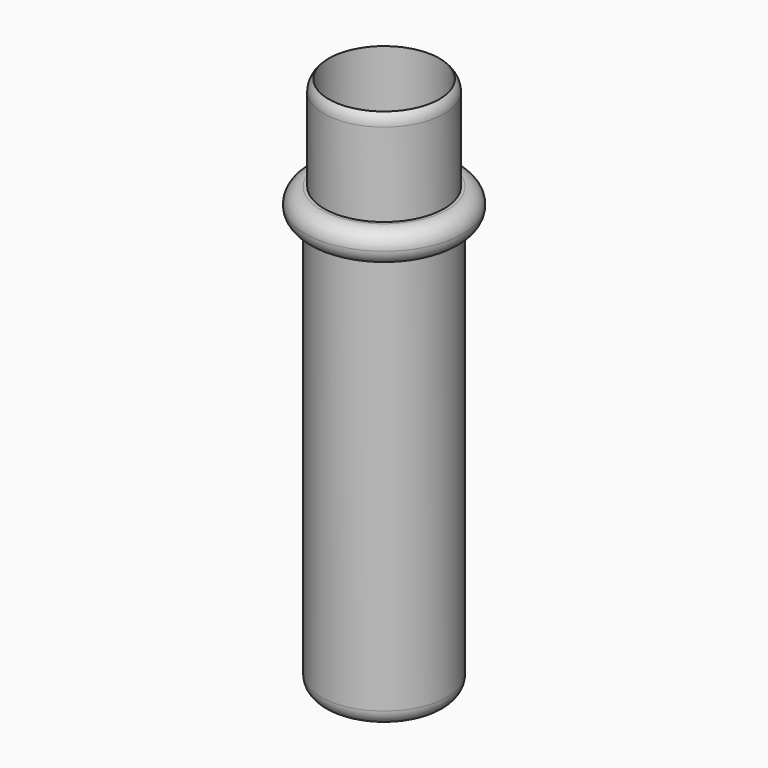
from build123d import *

# Parameters (mm, degrees)
F0_R      = 20
F0_R_2    = 17.5
F1_DEPTH  = 130
F2_R      = 25
F2_R_2    = 20
F2_R_3    = 17.5
F3_DEPTH  = 10
F4_R      = 19
F4_R_2    = 17.5
F5_DEPTH  = 30
F6_2_F1_R = 5
F6_2_F2_R = 4.9999


# Not quite as in the source:
# - a fillet or chamfer that OpenCascade refuses, or shapes differently, is made with other operations: its cross-section is extruded or revolved along the edge and cut away or added
# - a fillet or chamfer is up to 0.001 mm smaller than in the source, because OpenCascade refuses the exact size
# - a feature names something its author has since deleted; it is built from what else it names


with BuildPart() as f1:
    # F0 (on Top) → F1 (new body)
    with BuildSketch(Plane.XY):
        Circle(F0_R)
        Circle(F0_R_2, mode=Mode.SUBTRACT)
    extrude(amount=F1_DEPTH)

    # F6: fillet of radius 5 on 1 edges, made by hand

    # F6_s1 → F6_t2 (revolve, cut)
    with BuildSketch(Plane.XZ):
        with BuildLine():
            ThreePointArc((20, 4.3301270189), (19.3301270189, 1.8301270189), (17.5, 0))
            Line((17.5, 0), (20, 0))
            Line((20, 0), (20, 4.3301270189))
        make_face()
    revolve(axis=Axis((0, 0, 0), (0, 0, 1)), mode=Mode.SUBTRACT)


with BuildPart() as f3:
    # F2 (on face) → F3 (new body)
    with BuildSketch(Plane.XY.offset(130)):
        Circle(F2_R)
        Circle(F2_R_2, mode=Mode.SUBTRACT)
        Circle(F2_R_2)
        Circle(F2_R_3, mode=Mode.SUBTRACT)
    extrude(amount=F3_DEPTH)

    # F4 (on face) → F5 (join)
    with BuildSketch(Plane.XY.offset(140)):
        Circle(F4_R)
        Circle(F4_R_2, mode=Mode.SUBTRACT)
    extrude(amount=F5_DEPTH)

    # F6#2: fillet of radius 5 on 2 edges, made by hand

    # F6_2_f1
    f6_2_f1_edges = [f3.edges().sort_by_distance(p)[0] for p in [
        (-25, 0, 140),
    ]]
    fillet(f6_2_f1_edges, radius=F6_2_F1_R)

    # F6_2_f2 (radius 5 in the source; OpenCascade refuses exactly that, so slightly less here)
    f6_2_f2_edges = [f3.edges().sort_by_distance(p)[0] for p in [
        (-25, 0, 130),
    ]]
    fillet(f6_2_f2_edges, radius=F6_2_F2_R)

    # F7: fillet of radius 5 on 1 edges, made by hand

    # F7_s1 → F7_t2 (revolve, cut)
    with BuildSketch(Plane.XZ):
        with BuildLine():
            ThreePointArc((19, 166.4292857857), (18.6097722286, 168.3657774588), (17.5, 170))
            Line((17.5, 170), (19, 170))
            Line((19, 170), (19, 166.4292857857))
        make_face()
    revolve(axis=Axis((0, 0, 170), (0, 0, 1)), mode=Mode.SUBTRACT)


solid = Compound([f1.part, f3.part])
